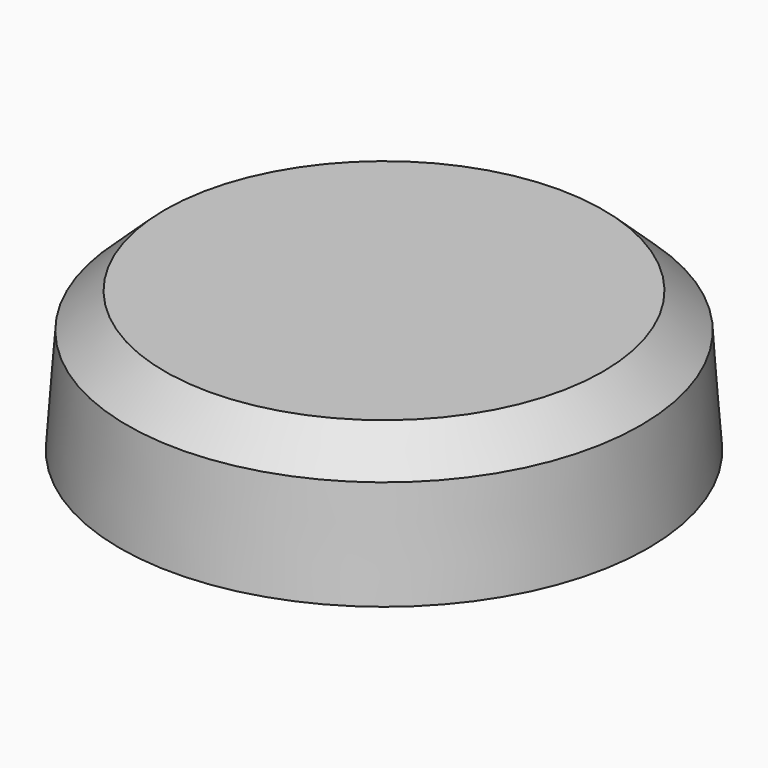
from build123d import *

# Parameters (mm, degrees)
F0_R     = 3.75
F1_DEPTH = 2
F1_TAPER = 4


# Not quite as in the source:
# - a fillet or chamfer that OpenCascade refuses, or shapes differently, is made with other operations: its cross-section is extruded or revolved along the edge and cut away or added


with BuildPart() as f1:
    # F0 (on Top) → F1 (new body)
    with BuildSketch(Plane.XY):
        Circle(F0_R)
    extrude(amount=F1_DEPTH, taper=F1_TAPER)

    # F2: chamfer of 0.5 on 1 edges, made by hand

    # F2_s1 → F2_t2 (revolve, cut)
    with BuildSketch(Plane.XZ):
        Polygon((3.645024613, 1.5012179749), (3.1101463761, 2), (3.6101463761, 2), align=None)
    revolve(axis=Axis((0, 0, 2), (0, 0, -1)), mode=Mode.SUBTRACT)


solid = f1.part
